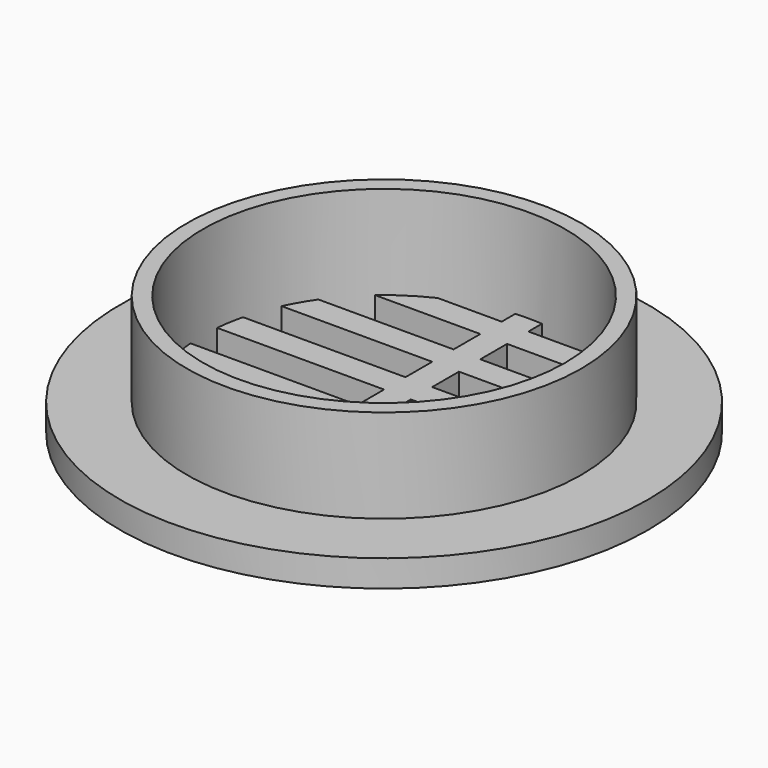
from build123d import *

# Parameters (mm, degrees)
F0_R      = 19.75
F1_DEPTH  = 2
F3_W      = 29.5
F3_H      = 2
F4_DEPTH  = 2
F5_R      = 14.75
F6_DEPTH  = 2
F9_R      = 14.75
F9_R_2    = 13.55
F10_DEPTH = 9
F11_W     = 2
F11_H     = 33.5
F12_DEPTH = 2


with BuildPart() as f1:
    # F0 (on Top) → F1 (new body)
    with BuildSketch(Plane.XY):
        Circle(F0_R)
    extrude(amount=F1_DEPTH)


with BuildPart() as f4:
    # F3 (on face) → F4 (new body, through all)
    with BuildSketch(Plane.XY.offset(2)):
        with Locations((0, -15.75)):
            Rectangle(F3_W, F3_H)
    extrude(amount=-F4_DEPTH)


with BuildPart() as f4b:
    # F3 (on face) → F4, piece 2 (new body, through all)
    with BuildSketch(Plane.XY.offset(2)):
        with Locations((0, -11.25)):
            Rectangle(F3_W, F3_H)
    extrude(amount=-F4_DEPTH)


with BuildPart() as f4c:
    # F3 (on face) → F4, piece 3 (new body, through all)
    with BuildSketch(Plane.XY.offset(2)):
        with Locations((0, -6.75)):
            Rectangle(F3_W, F3_H)
    extrude(amount=-F4_DEPTH)


with BuildPart() as f4d:
    # F3 (on face) → F4, piece 4 (new body, through all)
    with BuildSketch(Plane.XY.offset(2)):
        with Locations((0, -2.25)):
            Rectangle(F3_W, F3_H)
    extrude(amount=-F4_DEPTH)


with BuildPart() as f4e:
    # F3 (on face) → F4, piece 5 (new body, through all)
    with BuildSketch(Plane.XY.offset(2)):
        with Locations((0, 2.25)):
            Rectangle(F3_W, F3_H)
    extrude(amount=-F4_DEPTH)


with BuildPart() as f4f:
    # F3 (on face) → F4, piece 6 (new body, through all)
    with BuildSketch(Plane.XY.offset(2)):
        with Locations((0, 6.75)):
            Rectangle(F3_W, F3_H)
    extrude(amount=-F4_DEPTH)


with BuildPart() as f4g:
    # F3 (on face) → F4, piece 7 (new body, through all)
    with BuildSketch(Plane.XY.offset(2)):
        with Locations((0, 11.25)):
            Rectangle(F3_W, F3_H)
    extrude(amount=-F4_DEPTH)


with BuildPart() as f4h:
    # F3 (on face) → F4, piece 8 (new body, through all)
    with BuildSketch(Plane.XY.offset(2)):
        with Locations((0, 15.75)):
            Rectangle(F3_W, F3_H)
    extrude(amount=-F4_DEPTH)


with BuildPart() as f6:
    # F5 (on Top) → F6 (new body, through all)
    with BuildSketch(Plane.XY):
        Circle(F5_R)
    extrude(amount=F6_DEPTH)

    # F7: cut F4h, F4g, F4f, F4e, F4d, F4c, F4b, F4
    add(f4h.part, mode=Mode.SUBTRACT)
    add(f4g.part, mode=Mode.SUBTRACT)
    add(f4f.part, mode=Mode.SUBTRACT)
    add(f4e.part, mode=Mode.SUBTRACT)
    add(f4d.part, mode=Mode.SUBTRACT)
    add(f4c.part, mode=Mode.SUBTRACT)
    add(f4b.part, mode=Mode.SUBTRACT)
    add(f4.part, mode=Mode.SUBTRACT)


with BuildPart() as f1_1:
    add(f1.part)

    # F8: cut F6
    add(f6.part, mode=Mode.SUBTRACT)

    # F9 (on face) → F10 (join, through all)
    with BuildSketch(Plane.XY):
        Circle(F9_R)
        Circle(F9_R_2, mode=Mode.SUBTRACT)
    extrude(amount=F10_DEPTH)

    # F11 (on face) → F12 (join, through all)
    with BuildSketch(Plane.XY):
        Rectangle(F11_W, F11_H)
    extrude(amount=F12_DEPTH)


solid = f1_1.part
